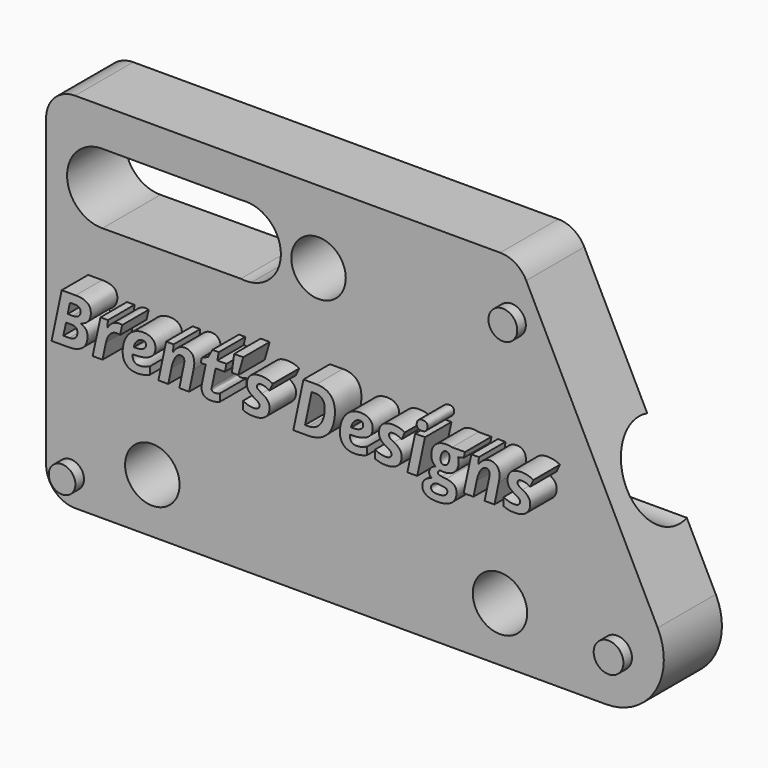
from build123d import *

# Parameters (mm, degrees)
F1_DEPTH      = 57.15
F3_DEPTH      = 10.922
F5_R          = 5.08
F6_R          = 2.54
F7_R          = 2.38125
F9_DEPTH      = 25.4
F10_TEXT_SIZE = 5.8699903699
F11_DEPTH     = 2.8956
F12_R         = 1.2594980203
F12_R_2       = 1.1648132834
F12_R_3       = 1.2985831896
F13_DEPTH     = 0.9398


# Not quite as in the source:
# - Text() gives the source's letters only with a copy of the font that has no kerning and outlines rounded to 1/6400 em; it was checked with that copy


with BuildPart() as f1:
    # F0 (on Right) → F1 (new body)
    with BuildSketch(Plane.YZ):
        with BuildLine():
            Line((0, 31.75), (0, 0))
            Line((0, 0), (6.35, 0))
            Line((6.35, 0), (6.35, 12.4206))
            ThreePointArc((6.35, 12.4206), (1.9434844301, 15.8765128344), (6.35, 19.3324256688))
            Line((6.35, 19.3324256688), (6.35, 31.75))
            Line((6.35, 31.75), (0, 31.75))
        make_face()
    extrude(amount=-F1_DEPTH)

    # F2 (on face) → F3 (cut)
    with BuildSketch(Plane.XZ):
        Polygon((0, 0), (0, 31.75), (-15.875, 31.75), align=None)
    extrude(amount=-F3_DEPTH, mode=Mode.SUBTRACT)

    # F5
    f5_edges = [f1.edges().sort_by_distance(p)[0] for p in [
        (0, 3.175, 0),
    ]]
    fillet(f5_edges, radius=F5_R)

    # F6
    f6_edges = [f1.edges().sort_by_distance(p)[0] for p in [
        (-57.15, 3.175, 31.75),
        (-57.15, 3.175, 0),
        (-15.875, 3.175, 31.75),
    ]]
    fillet(f6_edges, radius=F6_R)

    # F7 (on face) → F9 (cut)
    with BuildSketch(Plane.XZ):
        with Locations((-17.4625, 4.7625)):
            Circle(F7_R)
        with Locations((-47.8623919189, 4.7625)):
            Circle(F7_R)
        with Locations((-33.3283213405, 25.3990371708)):
            Circle(F7_R)
        with BuildLine():
            Line((-39.2121089515, 22.3787519439), (-40.1156129863, 22.37456125))
            ThreePointArc((-40.1156129863, 22.37456125), (-39.6637052843, 22.3430913652), (-39.2121089515, 22.3787519439))
        make_face()
        with BuildLine():
            Line((-52.2278059711, 22.3183816515), (-40.1156129863, 22.37456125))
            Line((-40.1156129863, 22.37456125), (-39.2121089515, 22.3787519439))
            ThreePointArc((-39.2121089515, 22.3787519439), (-36.6218148562, 25.469655661), (-39.3503951185, 28.4391941841))
            Line((-39.3503951185, 28.4391941841), (-40.0053722576, 28.4391941841))
            Line((-40.0053722576, 28.4391941841), (-52.2001155516, 28.4391941841))
            Line((-52.2001155516, 28.4391941841), (-52.3079621275, 28.4391941841))
            ThreePointArc((-52.3079621275, 28.4391941841), (-55.3144764234, 25.3388907418), (-52.2278059711, 22.3183816515))
        make_face()
        with BuildLine():
            Line((-40.0053722576, 28.4391941841), (-39.3503951185, 28.4391941841))
            ThreePointArc((-39.3503951185, 28.4391941841), (-39.677883688, 28.4567870936), (-40.0053722576, 28.4391941841))
        make_face()
        with BuildLine():
            ThreePointArc((-52.2001155516, 28.4391941841), (-52.2540388396, 28.4396692301), (-52.3079621275, 28.4391941841))
            Line((-52.3079621275, 28.4391941841), (-52.2001155516, 28.4391941841))
        make_face()
    extrude(amount=-F9_DEPTH, mode=Mode.SUBTRACT)

    # F10 (on face) → F11 (join)
    with BuildSketch(Plane.XZ):
        with Locations((-54.5059032738, 14.1365574673)):
            Text("Brent's Designs", F10_TEXT_SIZE, font='Open Sans', font_style=FontStyle.BOLDITALIC, text_align=(TextAlign.LEFT, TextAlign.BOTTOM))
    extrude(amount=F11_DEPTH)

    # F12 (on face) → F13 (join)
    with BuildSketch(Plane.XZ):
        with Locations((-16.4623521268, 26.8954206258)):
            Circle(F12_R)
        with Locations((-55.0012253225, 2.4740677327)):
            Circle(F12_R_2)
        with Locations((-7.2226105258, 4.3086726218)):
            Circle(F12_R_3)
    extrude(amount=F13_DEPTH)


solid = f1.part
